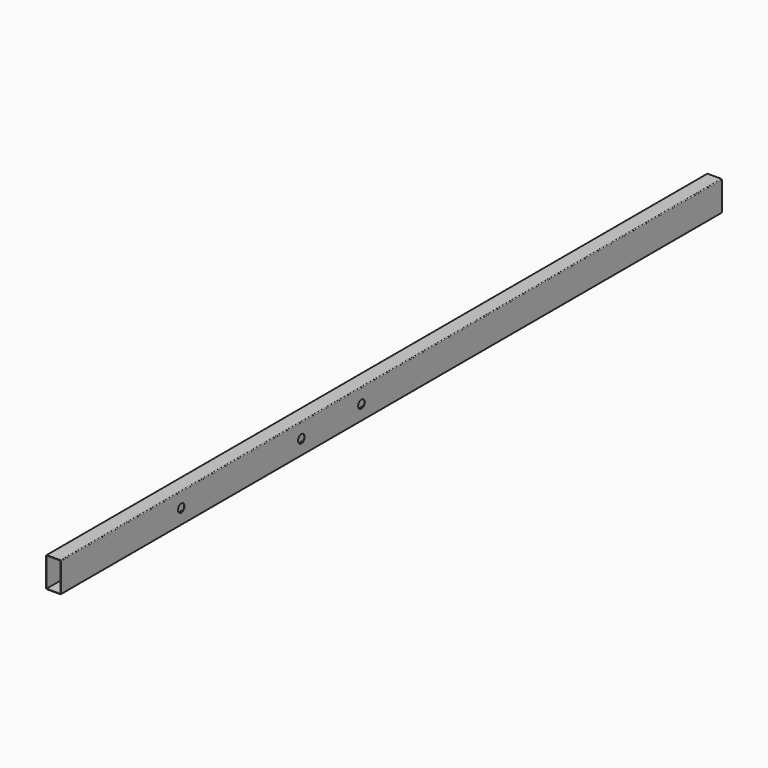
from build123d import *

# Parameters (mm, degrees)
F0_W     = 19
F0_H     = 39
F1_DEPTH = 550
F3_D     = 11
F3_DEPTH = 30
F3_TIP   = 3.3047334047


# Not quite as in the source:
# - a feature names something its author has since deleted; it is built from what else it names


with BuildPart() as f1:
    # F0 (on Front) → F1 (new body, symmetric)
    with BuildSketch(Plane.XZ):
        with BuildLine():
            Line((9, 20), (-9, 20))
            ThreePointArc((-9, 20), (-9.7071067812, 19.7071067812), (-10, 19))
            Line((-10, 19), (-10, -19))
            ThreePointArc((-10, -19), (-9.7071067812, -19.7071067812), (-9, -20))
            Line((-9, -20), (9, -20))
            ThreePointArc((9, -20), (9.7071067812, -19.7071067812), (10, -19))
            Line((10, -19), (10, 19))
            ThreePointArc((10, 19), (9.7071067812, 19.7071067812), (9, 20))
        make_face()
        Rectangle(F0_W, F0_H, mode=Mode.SUBTRACT)
    extrude(amount=F1_DEPTH, both=True)

    # F3
    with Locations(Plane.YZ.offset(10)):
        with Locations((-50, 0), (-150, 0), (-350, 0)):
            Hole(F3_D / 2, depth=F3_DEPTH)
            with Locations((0, 0, -(F3_DEPTH + F3_TIP / 2))):  # 118° drill point
                Cone(0, F3_D / 2, F3_TIP, mode=Mode.SUBTRACT)


solid = f1.part
